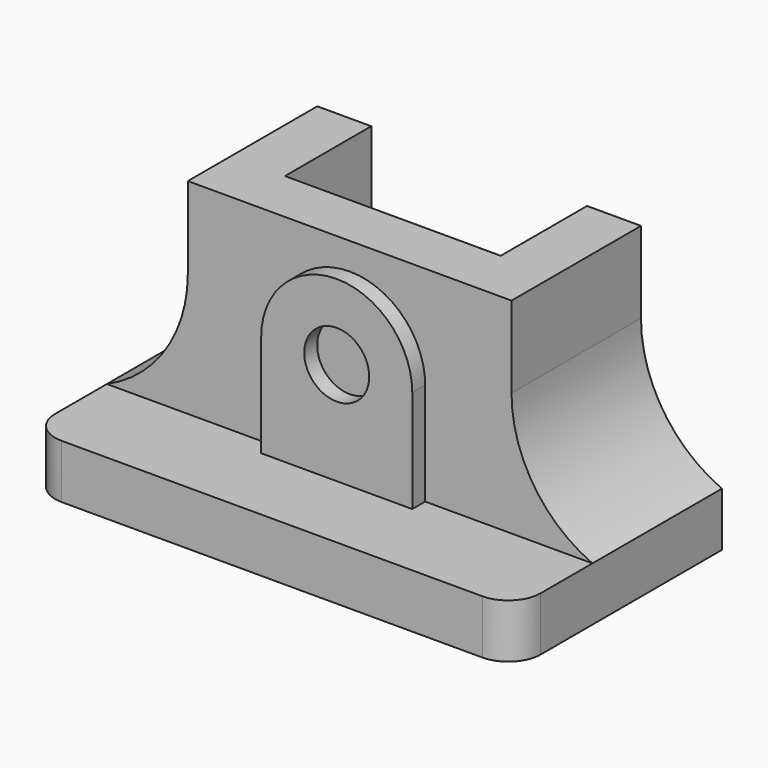
from build123d import *

# Parameters (mm, degrees)
F1_DEPTH    = 48
F2_DEPTH    = 10
F3_R        = 6.0205101074
F4_DEPTH    = 3
F5_T1_DEPTH = 30
F6_R        = 6


# Not quite as in the source:
# - a fillet or chamfer that OpenCascade refuses, or shapes differently, is made with other operations: its cross-section is extruded or revolved along the edge and cut away or added


with BuildPart() as f1:
    # F0 (on Top) → F1 (new body)
    with BuildSketch(Plane.XY):
        Polygon((20, 10), (0, 10), (-20, 10), (-20, 30), (-30, 30), (-30, 0), (0, 0), (30, 0), (30, 30), (20, 30), align=None)
    extrude(amount=F1_DEPTH)

    # F0 (on Top) → F2 (join)
    with BuildSketch(Plane.XY):
        Polygon((20, 10), (0, 10), (-20, 10), (-20, 30), (-30, 30), (-30, 0), (0, 0), (30, 0), (30, 30), (20, 30), align=None)
        Polygon((-30, 0), (-30, 30), (-45, 30), (-45, -18), (0, -18), (45, -18), (45, 30), (30, 30), (30, 0), (0, 0), align=None)
    extrude(amount=F2_DEPTH)

    # F3 (on Front) → F4 (join)
    with BuildSketch(Plane.XZ):
        with BuildLine():
            Line((14, 10), (14, 29))
            ThreePointArc((14, 29), (0, 43), (-14, 29))
            Line((-14, 29), (-14, 10))
            Line((-14, 10), (14, 10))
        make_face()
        with Locations((0, 29)):
            Circle(F3_R, mode=Mode.SUBTRACT)
    extrude(amount=F4_DEPTH)

    # F5: fillet of radius 25 on 2 edges, made by hand

    # F5_s2 → F5_t1 (join)
    with BuildSketch(Plane.XZ.offset(-30)):
        with BuildLine():
            ThreePointArc((30, 32.9128784748), (34.0834993366, 19.2198145372), (45, 10))
            Line((45, 10), (30, 10))
            Line((30, 10), (30, 32.9128784748))
        make_face()
        with BuildLine():
            ThreePointArc((-30, 32.9128784748), (-34.0834993366, 19.2198145372), (-45, 10))
            Line((-45, 10), (-30, 10))
            Line((-30, 10), (-30, 32.9128784748))
        make_face()
    extrude(amount=F5_T1_DEPTH)

    # F6
    f6_edges = [f1.edges().sort_by_distance(p)[0] for p in [
        (-45, -18, 5),
        (45, -18, 5),
    ]]
    fillet(f6_edges, radius=F6_R)


solid = f1.part
